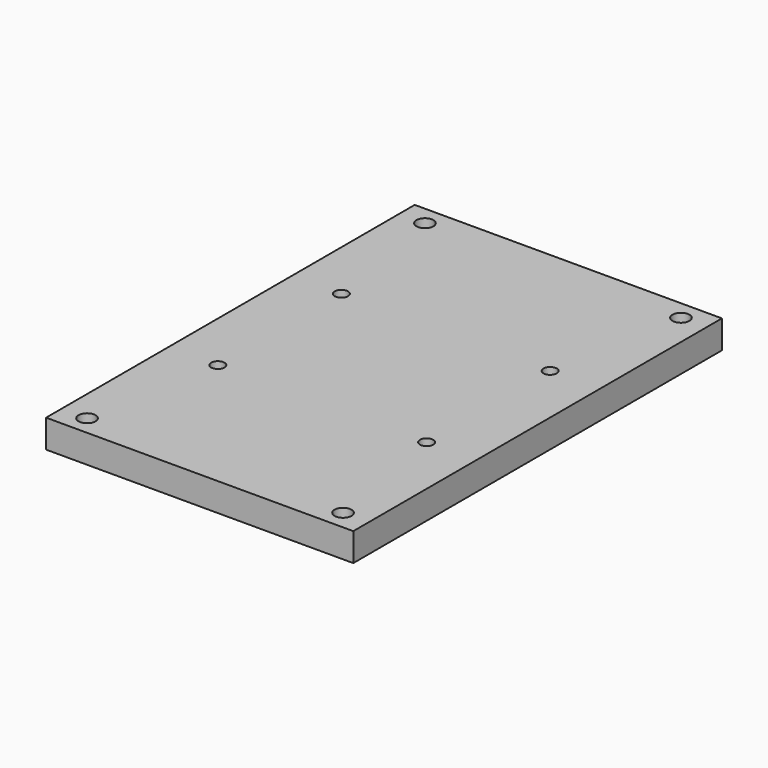
from build123d import *

# Parameters (mm, degrees)
F0_W     = 76.2
F0_H     = 114.3
F1_DEPTH = 6.985
F3_D     = 4.2
F6_D     = 3.3
F6_DEPTH = 12
F6_TIP   = 0.9914200214


# Not quite as in the source:
# - a pattern or mirror of a feature is missing from the dataset's text; its kind, count and spacing are read off the source's solid
# - a feature names something its author has since deleted; it is built from what else it names


with BuildPart() as f1:
    # F0 (on Top) → F1 (new body)
    with BuildSketch(Plane.XY):
        Rectangle(F0_W, F0_H)
    extrude(amount=F1_DEPTH)

    # F3 (through all)
    with Locations(Plane.XY.offset(6.985)):
        with Locations((-31.75, 52.3875), (31.75, 52.3875), (31.75, -52.3875), (-31.75, -52.3875)):
            Hole(F3_D / 2)

    # F6
    with Locations(Plane.XY.offset(6.985)):
        with Locations((-25.9, -19.15), (25.9, -19.15)):
            f6 = Hole(F6_D / 2, depth=F6_DEPTH)
            with Locations((0, 0, -(F6_DEPTH + F6_TIP / 2))):  # 118° drill point
                Cone(0, F6_D / 2, F6_TIP, mode=Mode.SUBTRACT)

    # F6_copies: F6 across plane
    add(f6.mirror(Plane.ZX), mode=Mode.SUBTRACT)


solid = f1.part
